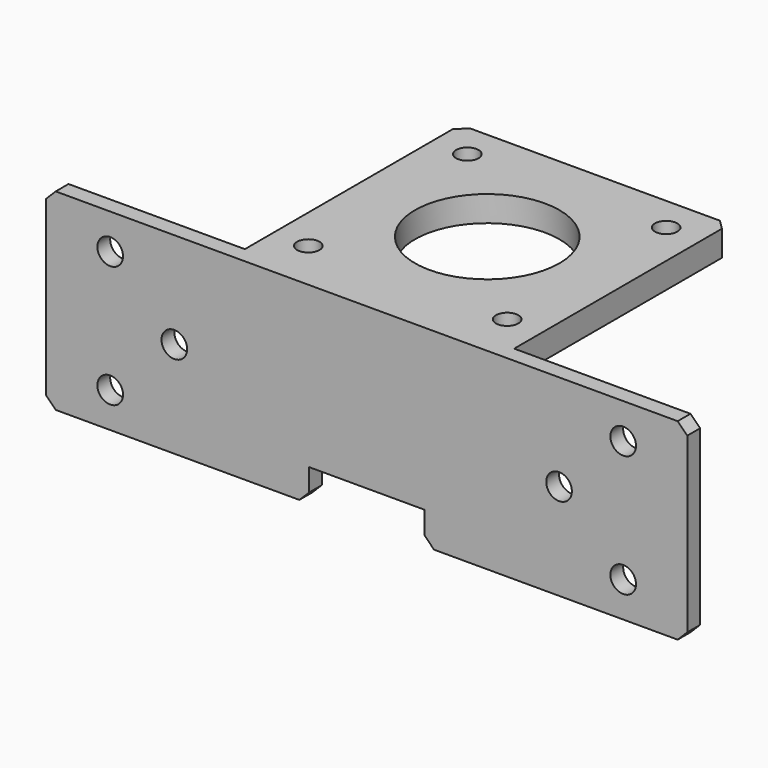
from build123d import *

# Parameters (mm, degrees)
F0_W     = 42
F0_H     = 42
F0_R     = 1.75
F0_R_2   = 11.25
F1_DEPTH = 4
F2_R     = 2
F2_W     = 42
F2_H     = 4
F3_DEPTH = 2.5
F4_SIZE  = 1.5


# Not quite as in the source:
# - a feature names something its author has since deleted; it is built from what else it names


with BuildPart() as f1:
    # F0 (on Top) → F1 (new body)
    with BuildSketch(Plane.XY):
        Rectangle(F0_W, F0_H)
        with Locations((-15.5, -15.5)):
            Circle(F0_R, mode=Mode.SUBTRACT)
        with Locations((15.5, -15.5)):
            Circle(F0_R, mode=Mode.SUBTRACT)
        with Locations((-15.5, 15.5)):
            Circle(F0_R, mode=Mode.SUBTRACT)
        Circle(F0_R_2, mode=Mode.SUBTRACT)
        with Locations((15.5, 15.5)):
            Circle(F0_R, mode=Mode.SUBTRACT)
    extrude(amount=-F1_DEPTH)

    # F2 (on face) → F3 (join)
    with BuildSketch(Plane.XZ.offset(21)):
        Polygon((50, -30), (50, 0), (21, 0), (21, -4), (-21, -4), (-21, 0), (-50, 0), (-50, -30), (-9, -30), (-9, -25), (9, -25), (9, -30), align=None)
        with Locations((-40, -24.5)):
            Circle(F2_R, mode=Mode.SUBTRACT)
        with Locations((40, -24.5)):
            Circle(F2_R, mode=Mode.SUBTRACT)
        with Locations((-30, -15)):
            Circle(F2_R, mode=Mode.SUBTRACT)
        with Locations((-40, -5.5)):
            Circle(F2_R, mode=Mode.SUBTRACT)
        with Locations((30, -15)):
            Circle(F2_R, mode=Mode.SUBTRACT)
        with Locations((40, -5.5)):
            Circle(F2_R, mode=Mode.SUBTRACT)
        with Locations((0, -2)):
            Rectangle(F2_W, F2_H)
    extrude(amount=F3_DEPTH)

    # F4
    f4_edges = [f1.edges().sort_by_distance(p)[0] for p in [
        (-21, 21, -2),
        (21, 21, -2),
        (-50, -22.25, 0),
        (-50, -22.25, -30),
        (50, -22.25, -30),
        (50, -22.25, 0),
        (-9, -22.25, -30),
        (9, -22.25, -30),
    ]]
    chamfer(f4_edges, length=F4_SIZE)


solid = f1.part
